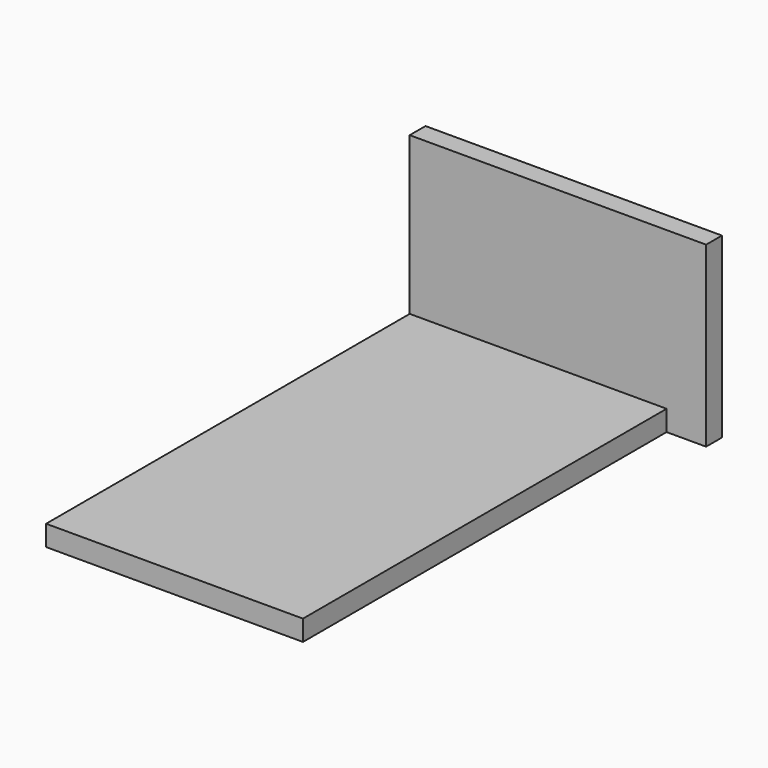
from build123d import *

# Parameters (mm, degrees)
F0_W     = 330.2
F0_H     = 26.4121327996
F1_DEPTH = 609.6
F2_W     = 381
F2_H     = 228.6
F3_DEPTH = 25.4


# Not quite as in the source:
# - a feature names something its author has since deleted; it is built from what else it names


with BuildPart() as f1:
    # F0 (on Front) → F1 (new body)
    with BuildSketch(Plane.XZ):
        with Locations((0, -113.7939336002)):
            Rectangle(F0_W, F0_H)
    extrude(amount=-F1_DEPTH)

    # F2 (on face) → F3 (join)
    with BuildSketch(Plane(origin=(0, 609.6, 0), x_dir=(-1, 0, 0), z_dir=(0, 1, 0))):
        with Locations((-25.4, -12.7)):
            Rectangle(F2_W, F2_H)
    extrude(amount=-F3_DEPTH)


solid = f1.part
